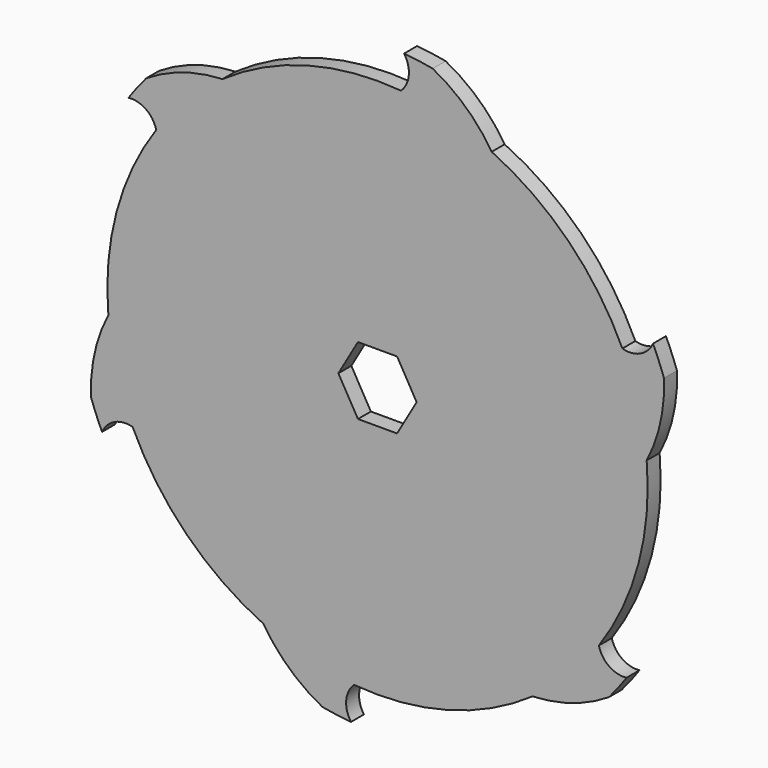
from build123d import *

# Parameters (mm, degrees)
F0_R            = 50.00625
F1_DEPTH        = 1.3335
F3_DEPTH        = 25.4
F3_DEPTH_BACK   = 25.4
F3_COPIES_COUNT = 6


# Not quite as in the source:
# - a pattern or mirror of a feature is missing from the dataset's text; its kind, count and spacing are read off the source's solid


with BuildPart() as f1:
    # F0 (on Front) → F1 (new body, symmetric)
    with BuildSketch(Plane.XZ):
        Circle(F0_R)
        Polygon((-6.4378019116, 0), (-3.2189009558, 5.5753), (3.2189009558, 5.5753), (6.4378019116, 0), (3.2189009558, -5.5753), (-3.2189009558, -5.5753), align=None, mode=Mode.SUBTRACT)
    extrude(amount=F1_DEPTH, both=True)

    # F2 (on Front) → F3 (cut, two sides)
    with BuildSketch(Plane.XZ) as f3_sk:
        with BuildLine():
            ThreePointArc((-25.4954725958, 36.4113083686), (-11.5045065548, 42.9354029785), (3.8740727651, 44.2808543302))
            ThreePointArc((3.8740727651, 44.2808543302), (5.1530874963, 46.9576920269), (4.3583318608, 49.8159611215))
            ThreePointArc((4.3583318608, 49.8159611215), (-18.9514344885, 46.275999934), (-38.0483910305, 32.4491136867))
            ThreePointArc((-38.0483910305, 32.4491136867), (-32.0330640833, 35.25752325), (-25.4954725958, 36.4113083686))
        make_face()
    f3 = extrude(amount=-F3_DEPTH, mode=Mode.SUBTRACT) + extrude(f3_sk.sketch, amount=F3_DEPTH_BACK, mode=Mode.SUBTRACT)

    # F3_copies: F3 ×6 about axis
    f3_copies_axis = Axis((0, 0, 0), (0, 1, 0))
    for i in range(1, F3_COPIES_COUNT):
        add(f3.rotate(f3_copies_axis, i * 360 / F3_COPIES_COUNT), mode=Mode.SUBTRACT)


solid = f1.part
